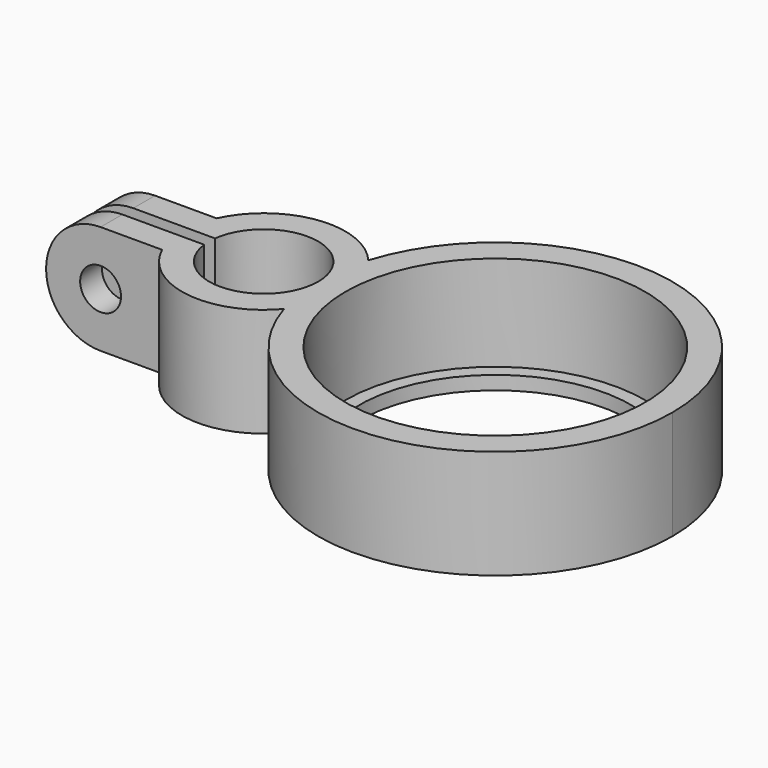
from build123d import *

# Parameters (mm, degrees)
F1_DEPTH = 1
F2_DEPTH = 8
F4_R     = 3.99999
F5_DEPTH = 5


# Not quite as in the source:
# - a fillet or chamfer is up to 0.001 mm smaller than in the source, because OpenCascade refuses the exact size


with BuildPart() as f1:
    # F0 (on Top) → F1 (new body)
    with BuildSketch(Plane.XY):
        with BuildLine():
            ThreePointArc((-24.6977130771, 2.8230095394), (-35.6977130771, 13.8230095394), (-46.6977130771, 2.8230095394))
            ThreePointArc((-46.6977130771, 2.8230095394), (-35.6977130771, -8.1769904606), (-24.6977130771, 2.8230095394))
        make_face()
        with BuildLine():
            ThreePointArc((-45.6977130771, 2.8230095394), (-35.6977130771, 12.8230095394), (-25.6977130771, 2.8230095394))
            ThreePointArc((-25.6977130771, 2.8230095394), (-35.6977130771, -7.1769904606), (-45.6977130771, 2.8230095394))
        make_face(mode=Mode.SUBTRACT)
    extrude(amount=F1_DEPTH)

    # F0 (on Top) → F2 (join)
    with BuildSketch(Plane.XY):
        with BuildLine():
            ThreePointArc((-58.6768434486, 3.3230095394), (-58.5012596634, 4.3457856294), (-58.1520691344, 5.3230095394))
            Line((-58.1520691344, 5.3230095394), (-66.6663400437, 5.3230095394))
            Line((-66.6663400437, 5.3230095394), (-66.6663400437, 3.3230095394))
            Line((-66.6663400437, 3.3230095394), (-61.1977130771, 3.3230095394))
            Line((-61.1977130771, 3.3230095394), (-58.6768434486, 3.3230095394))
        make_face()
        with BuildLine():
            Line((-66.6663400437, 0.3230095394), (-58.1520691344, 0.3230095394))
            ThreePointArc((-58.1520691344, 0.3230095394), (-58.5012596634, 1.3002334494), (-58.6768434486, 2.3230095394))
            Line((-58.6768434486, 2.3230095394), (-61.1977130771, 2.3230095394))
            Line((-61.1977130771, 2.3230095394), (-66.6663400437, 2.3230095394))
            Line((-66.6663400437, 2.3230095394), (-66.6663400437, 0.3230095394))
        make_face()
        with BuildLine():
            Line((-58.6768434486, 3.3230095394), (-56.6663400437, 3.3230095394))
            Line((-56.6663400437, 3.3230095394), (-56.6663400437, 5.3230095394))
            Line((-56.6663400437, 5.3230095394), (-58.1520691344, 5.3230095394))
            ThreePointArc((-58.1520691344, 5.3230095394), (-58.5012596634, 4.3457856294), (-58.6768434486, 3.3230095394))
        make_face()
        with BuildLine():
            Line((-56.6663400437, 0.3230095394), (-56.6663400437, 2.3230095394))
            Line((-56.6663400437, 2.3230095394), (-58.6768434486, 2.3230095394))
            ThreePointArc((-58.6768434486, 2.3230095394), (-58.5012596634, 1.3002334494), (-58.1520691344, 0.3230095394))
            Line((-58.1520691344, 0.3230095394), (-56.6663400437, 0.3230095394))
        make_face()
        with BuildLine():
            ThreePointArc((-56.6663400437, 3.3230095394), (-52.4472214269, 6.8151585763), (-48.6977130771, 2.8230095394))
            ThreePointArc((-48.6977130771, 2.8230095394), (-48.5498129284, 4.7783942616), (-48.109477783, 6.6892864159))
            ThreePointArc((-48.109477783, 6.6892864159), (-53.5065513921, 8.768241291), (-58.1520691344, 5.3230095394))
            Line((-58.1520691344, 5.3230095394), (-56.6663400437, 5.3230095394))
            Line((-56.6663400437, 5.3230095394), (-56.6663400437, 3.3230095394))
        make_face()
        with BuildLine():
            ThreePointArc((-48.109477783, -1.0432673371), (-48.5498129284, 0.8676248172), (-48.6977130771, 2.8230095394))
            ThreePointArc((-48.6977130771, 2.8230095394), (-52.4472214269, -1.1691394976), (-56.6663400437, 2.3230095394))
            Line((-56.6663400437, 2.3230095394), (-56.6663400437, 0.3230095394))
            Line((-56.6663400437, 0.3230095394), (-58.1520691344, 0.3230095394))
            ThreePointArc((-58.1520691344, 0.3230095394), (-53.5065513921, -3.1222222122), (-48.109477783, -1.0432673371))
        make_face()
        with BuildLine():
            ThreePointArc((-48.109477783, 6.6892864159), (-47.0616944573, 4.8809925611), (-46.6977130771, 2.8230095394))
            ThreePointArc((-46.6977130771, 2.8230095394), (-47.0616944573, 0.7650265177), (-48.109477783, -1.0432673371))
            ThreePointArc((-48.109477783, -1.0432673371), (-33.7423283549, -10.0290903119), (-22.6977130771, 2.8230095394))
            ThreePointArc((-22.6977130771, 2.8230095394), (-33.7423283549, 15.6751093907), (-48.109477783, 6.6892864159))
        make_face()
        with BuildLine():
            ThreePointArc((-24.6977130771, 2.8230095394), (-35.6977130771, -8.1769904606), (-46.6977130771, 2.8230095394))
            ThreePointArc((-46.6977130771, 2.8230095394), (-35.6977130771, 13.8230095394), (-24.6977130771, 2.8230095394))
        make_face(mode=Mode.SUBTRACT)
        with BuildLine():
            ThreePointArc((-48.109477783, -1.0432673371), (-47.0616944573, 0.7650265177), (-46.6977130771, 2.8230095394))
            Line((-46.6977130771, 2.8230095394), (-48.6977130771, 2.8230095394))
            ThreePointArc((-48.6977130771, 2.8230095394), (-48.5498129284, 0.8676248172), (-48.109477783, -1.0432673371))
        make_face()
        with BuildLine():
            Line((-48.6977130771, 2.8230095394), (-46.6977130771, 2.8230095394))
            ThreePointArc((-46.6977130771, 2.8230095394), (-47.0616944573, 4.8809925611), (-48.109477783, 6.6892864159))
            ThreePointArc((-48.109477783, 6.6892864159), (-48.5498129284, 4.7783942616), (-48.6977130771, 2.8230095394))
        make_face()
    extrude(amount=F2_DEPTH)

    # F4 (radius 4 in the source; OpenCascade refuses exactly that, so slightly less here)
    f4_edges = [f1.edges().sort_by_distance(p)[0] for p in [
        (-66.66634, 4.32301, 8),
        (-66.66634, 1.32301, 8),
        (-66.66634, 4.32301, 0),
        (-66.66634, 1.32301, 0),
    ]]
    fillet(f4_edges, radius=F4_R)

    # F3 (on face) → F5 (cut)
    with BuildSketch(Plane.XZ.offset(-0.3230095394)):
        with BuildLine():
            Line((-64.1663400437, 4), (-61.1663400437, 4))
            ThreePointArc((-61.1663400437, 4), (-62.6663400437, 5.5), (-64.1663400437, 4))
        make_face()
        with BuildLine():
            ThreePointArc((-64.1663400437, 4), (-62.6663400437, 2.5), (-61.1663400437, 4))
            Line((-61.1663400437, 4), (-64.1663400437, 4))
        make_face()
    extrude(amount=-F5_DEPTH, mode=Mode.SUBTRACT)


solid = f1.part
